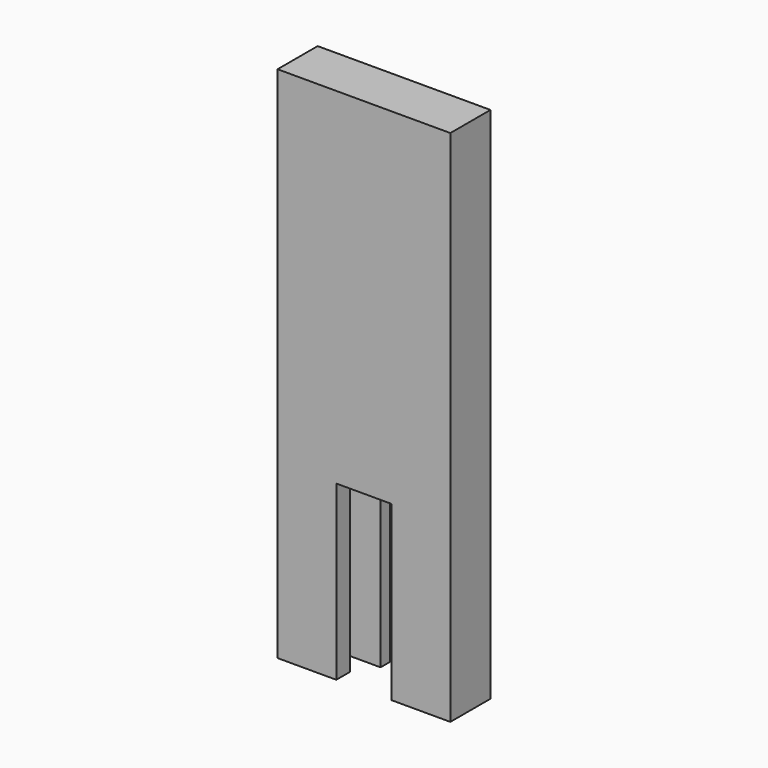
from build123d import *

# Parameters (mm, degrees)
F0_W      = 50
F0_H      = 150
F1_DEPTH  = 3.5
F3_DEPTH  = 6
F4_DEPTH  = 25
F5_W      = 50
F5_H      = 150
F6_DEPTH  = 5
F7_R      = 16
F7_R_2    = 4
F8_DEPTH  = 1
F9_DEPTH  = 5
F10_DEPTH = 10
F11_W     = 16
F11_H     = 50
F12_DEPTH = 6.1


with BuildPart() as f1:
    # F0 (on Front) → F1 (new body)
    with BuildSketch(Plane.XZ):
        Rectangle(F0_W, F0_H)
    extrude(amount=F1_DEPTH)

    # F2 (on face) → F3 (join)
    with BuildSketch(Plane.XZ.offset(3.5)):
        with BuildLine():
            Line((-13, 68), (13, 68))
            ThreePointArc((13, 68), (16.5355339059, 66.5355339059), (18, 63))
            Line((18, 63), (18, -68))
            Line((18, -68), (18, -75))
            Line((18, -75), (25, -75))
            Line((25, -75), (25, 75))
            Line((25, 75), (-25, 75))
            Line((-25, 75), (-25, -75))
            Line((-25, -75), (-18, -75))
            Line((-18, -75), (-18, -68))
            Line((-18, -68), (-18, 63))
            ThreePointArc((-18, 63), (-16.5355339059, 66.5355339059), (-13, 68))
        make_face()
    extrude(amount=F3_DEPTH)

    # F2 (on face) → F4 (cut)
    with BuildSketch(Plane.XZ.offset(3.5)):
        with BuildLine():
            Line((-4, -75), (4, -75))
            Line((4, -75), (4, 52))
            ThreePointArc((4, 52), (2.8284271247, 54.8284271247), (0, 56))
            ThreePointArc((0, 56), (-2.8284271247, 54.8284271247), (-4, 52))
            Line((-4, 52), (-4, -75))
        make_face()
    extrude(amount=-F4_DEPTH, mode=Mode.SUBTRACT)

    # F5 (on face) → F6 (join)
    with BuildSketch(Plane.XZ.offset(9.5)):
        Rectangle(F5_W, F5_H)
    extrude(amount=F6_DEPTH)

    # F11 (on face) → F12 (cut)
    with BuildSketch(Plane.XZ.offset(14.5)):
        with Locations((0, -50)):
            Rectangle(F11_W, F11_H)
    extrude(amount=-F12_DEPTH, mode=Mode.SUBTRACT)


with BuildPart() as f8:
    # F7 (on Front) → F8 (new body)
    with BuildSketch(Plane.XZ):
        with BuildLine():
            ThreePointArc((-18, -15), (-17.1213203436, -17.1213203436), (-15, -18))
            Line((-15, -18), (15, -18))
            ThreePointArc((15, -18), (17.1213203436, -17.1213203436), (18, -15))
            Line((18, -15), (18, 15))
            ThreePointArc((18, 15), (17.1213203436, 17.1213203436), (15, 18))
            Line((15, 18), (-15, 18))
            ThreePointArc((-15, 18), (-17.1213203436, 17.1213203436), (-18, 15))
            Line((-18, 15), (-18, -15))
        make_face()
        Circle(F7_R, mode=Mode.SUBTRACT)
        Circle(F7_R)
        Circle(F7_R_2, mode=Mode.SUBTRACT)
        Circle(F7_R_2)
    extrude(amount=F8_DEPTH)

    # F7 (on Front) → F9 (join)
    with BuildSketch(Plane.XZ):
        with BuildLine():
            ThreePointArc((-18, -15), (-17.1213203436, -17.1213203436), (-15, -18))
            Line((-15, -18), (15, -18))
            ThreePointArc((15, -18), (17.1213203436, -17.1213203436), (18, -15))
            Line((18, -15), (18, 15))
            ThreePointArc((18, 15), (17.1213203436, 17.1213203436), (15, 18))
            Line((15, 18), (-15, 18))
            ThreePointArc((-15, 18), (-17.1213203436, 17.1213203436), (-18, 15))
            Line((-18, 15), (-18, -15))
        make_face()
        Circle(F7_R, mode=Mode.SUBTRACT)
    extrude(amount=F9_DEPTH)

    # F7 (on Front) → F10 (join)
    with BuildSketch(Plane.XZ):
        Circle(F7_R_2)
    extrude(amount=-F10_DEPTH)


solid = Compound([f1.part, f8.part])
